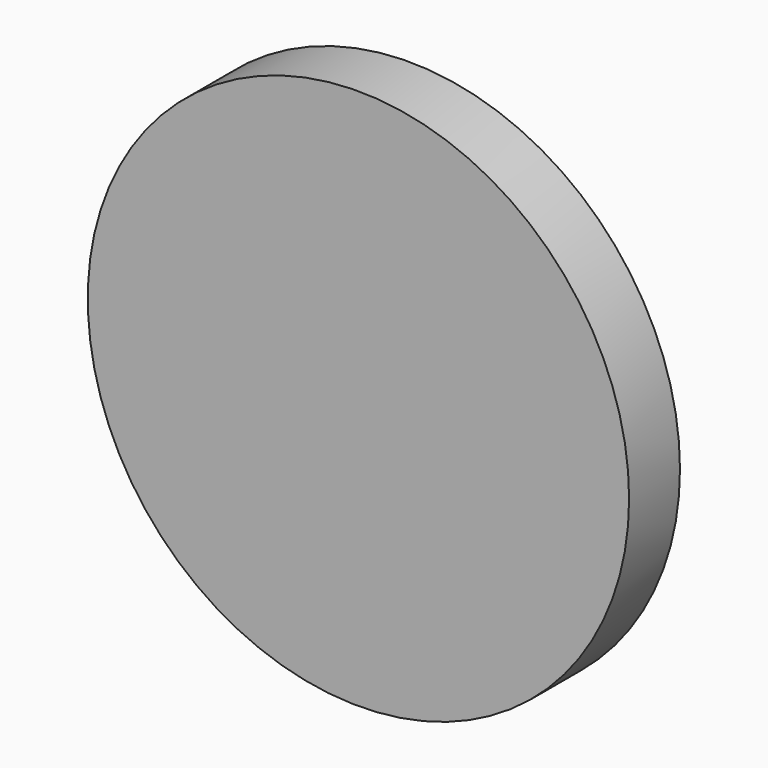
from build123d import *

# Parameters (mm, degrees)
F2_R     = 108.1201548103
F3_DEPTH = 25.4


# Not quite as in the source:
# - the program builds the solid bodies; features that only make, move or delete a surface that nothing else refers to are left out


with BuildPart() as f3:
    # F2 (on Front) → F3 (new body)
    with BuildSketch(Plane.XZ):
        with Locations((0, -82.8203931451)):
            Circle(F2_R)
    extrude(amount=F3_DEPTH)


solid = f3.part
